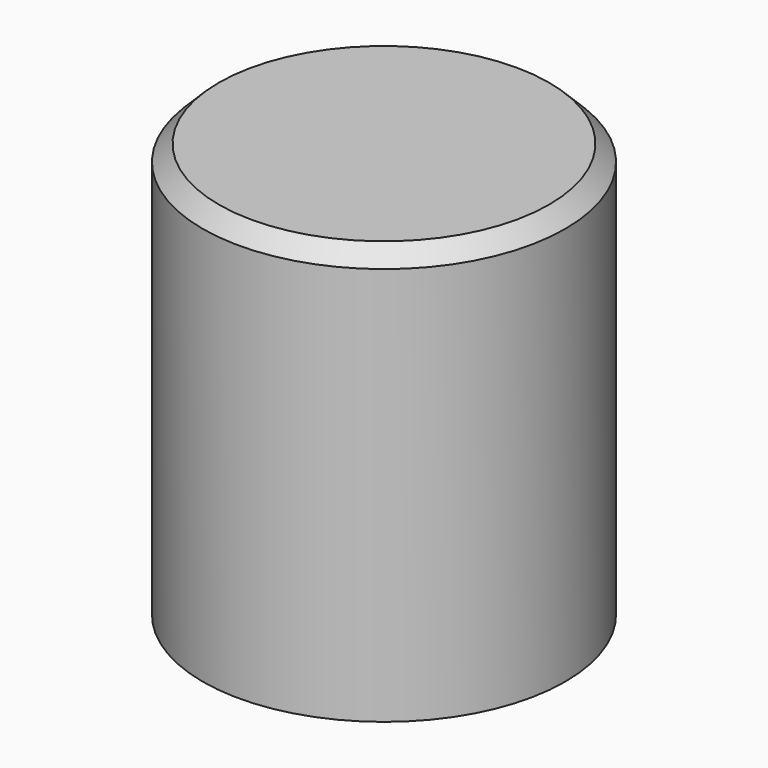
from build123d import *

# Parameters (mm, degrees)
F0_R     = 22.5074090386
F1_DEPTH = 49.5
F2_DEPTH = 2
F3_SIZE  = 2
F4_T     = -2.5


with BuildPart() as f1:
    # F0 (on Top) → F1 (new body)
    with BuildSketch(Plane.XY):
        Circle(F0_R)
    extrude(amount=F1_DEPTH)

    # F2 (add): a face of the model
    f2_faces = [f1.faces().sort_by_distance(p)[0] for p in [
        (0, 0, 49.5),
    ]]
    extrude(f2_faces, amount=F2_DEPTH)

    # F3
    f3_edges = [f1.edges().sort_by_distance(p)[0] for p in [
        (-22.507409, 0, 51.5),
    ]]
    chamfer(f3_edges, length=F3_SIZE)

    # F4
    f4_openings = [f1.faces().sort_by_distance(p)[0] for p in [
        (0, 0, 0),
    ]]
    offset(amount=F4_T, openings=f4_openings)


solid = f1.part
